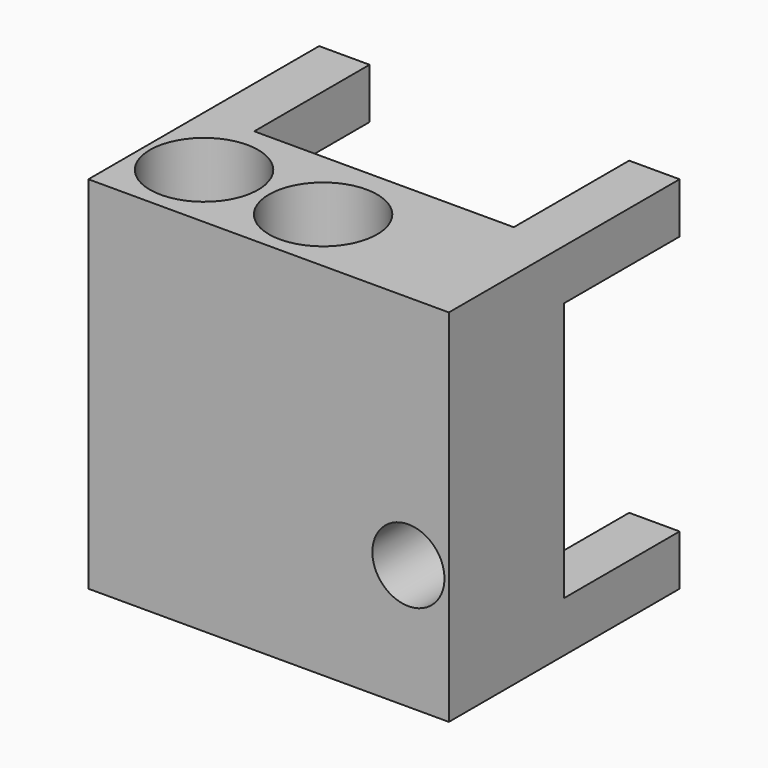
from build123d import *

# Parameters (mm, degrees)
F0_W     = 31.75
F0_H     = 63.5
F1_DEPTH = 25.4
F4_D     = 12.7
F4_DEPTH = 25.4
F4_TIP   = 3.8154649308
F5_W     = 8.89
F5_H     = 8.89
F6_DEPTH = 25.4
F7_D     = 19.05
F7_DEPTH = 50.8
F7_TIP   = 5.7231973962


# Not quite as in the source:
# - a feature names something its author has since deleted; it is built from what else it names


with BuildPart() as f1:
    # F0 (on Front) → F1 (new body)
    with BuildSketch(Plane.XZ):
        with Locations((15.875, 31.75)):
            Rectangle(F0_W, F0_H)
        with Locations((-15.875, 31.75)):
            Rectangle(F0_W, F0_H)
    extrude(amount=-F1_DEPTH)

    # F4
    with Locations(Plane.XZ):
        with Locations((24.6206466109, 21.9729263335)):
            Hole(F4_D / 2, depth=F4_DEPTH)
            with Locations((0, 0, -(F4_DEPTH + F4_TIP / 2))):  # 118° drill point
                Cone(0, F4_D / 2, F4_TIP, mode=Mode.SUBTRACT)

    # F5 (on face) → F6 (join)
    with BuildSketch(Plane(origin=(0, 25.4, 0), x_dir=(-1, 0, 0), z_dir=(0, 1, 0))):
        with Locations((-27.305, 59.055)):
            Rectangle(F5_W, F5_H)
        with Locations((27.305, 59.055)):
            Rectangle(F5_W, F5_H)
        with Locations((-27.305, 4.445)):
            Rectangle(F5_W, F5_H)
        with Locations((27.305, 4.445)):
            Rectangle(F5_W, F5_H)
    extrude(amount=F6_DEPTH)

    # F7
    with Locations(Plane.XY.offset(63.5)):
        with Locations((-21.082, 12.1284499764), (0, 11.9907837361)):
            Hole(F7_D / 2, depth=F7_DEPTH)
            with Locations((0, 0, -(F7_DEPTH + F7_TIP / 2))):  # 118° drill point
                Cone(0, F7_D / 2, F7_TIP, mode=Mode.SUBTRACT)


solid = f1.part
